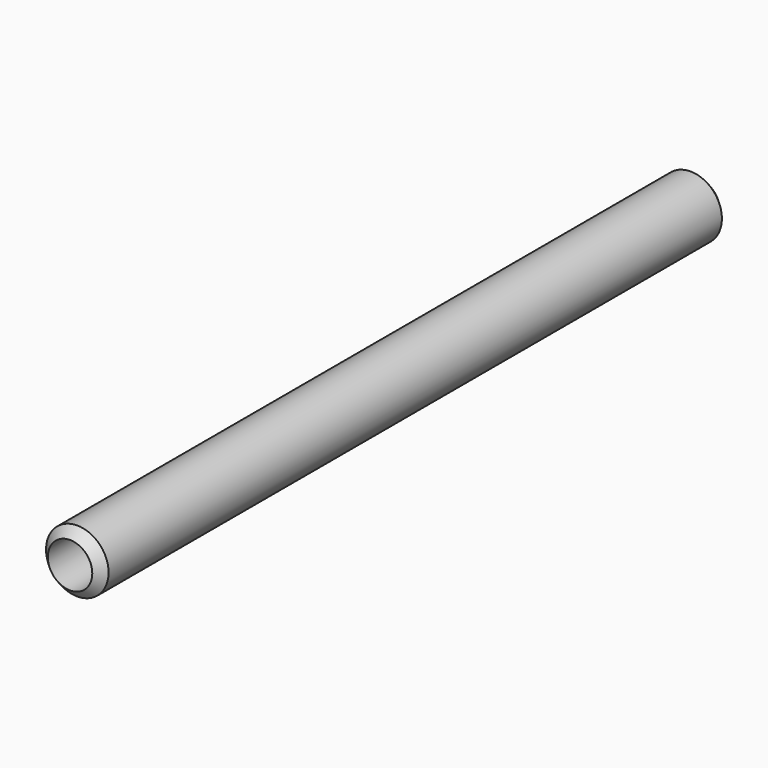
from build123d import *

# Parameters (mm, degrees)
F0_R     = 30.1625
F1_DEPTH = 762
F3_D     = 42.8498


# Not quite as in the source:
# - a fillet or chamfer that OpenCascade refuses, or shapes differently, is made with other operations: its cross-section is extruded or revolved along the edge and cut away or added


with BuildPart() as f1:
    # F0 (on Front) → F1 (new body)
    with BuildSketch(Plane.XZ):
        Circle(F0_R)
    extrude(amount=F1_DEPTH)

    # F3 (through all)
    with Locations(Plane.XZ.offset(762)):
        with Locations((0, 0)):
            Hole(F3_D / 2)

    # F4: chamfer of 11.38682 on 2 edges, made by hand

    # F4_s1 → F4_t2 (revolve, cut)
    with BuildSketch(Plane.XY):
        Polygon((30.1625, -750.61318), (18.77568, -762), (30.1625, -762), align=None)
    revolve(axis=Axis((0, -762, 0), (0, -1, 0)), mode=Mode.SUBTRACT)

    # F4_s3 → F4_t4 (revolve, cut)
    with BuildSketch(Plane.XY):
        Polygon((30.1625, -11.38682), (18.77568, 0), (30.1625, 0), align=None)
    revolve(axis=Axis((0, 0, 0), (0, -1, 0)), mode=Mode.SUBTRACT)


solid = f1.part
